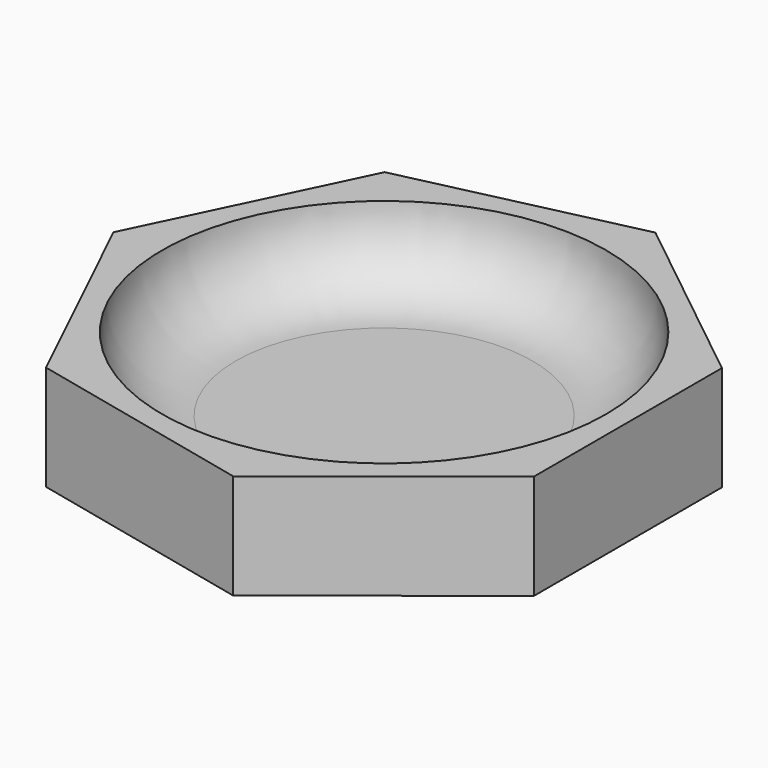
from build123d import *

# Parameters (mm, degrees)
F1_DEPTH = 25.4
F2_R     = 53.6748278482
F3_DEPTH = 17.78
F4_R     = 17.77999


# Not quite as in the source:
# - a fillet or chamfer is up to 0.001 mm smaller than in the source, because OpenCascade refuses the exact size


with BuildPart() as f1:
    # F0 (on Top) → F1 (new body)
    with BuildSketch(Plane.XY):
        Polygon((58.9595362544, -28.3934161968), (58.9595362544, 28.3934161968), (14.5618028995, 63.799427074), (-40.8012650454, 51.1631680934), (-65.440148217, 0), (-40.8012650454, -51.1631680934), (14.5618028995, -63.799427074), align=None)
    extrude(amount=F1_DEPTH)

    # F2 (on face) → F3 (cut)
    with BuildSketch(Plane.XY.offset(25.4)):
        Circle(F2_R)
    extrude(amount=-F3_DEPTH, mode=Mode.SUBTRACT)

    # F4 (radius 17.78 in the source; OpenCascade refuses exactly that, so slightly less here)
    f4_edges = [f1.edges().sort_by_distance(p)[0] for p in [
        (-53.674828, 0, 7.62),
    ]]
    fillet(f4_edges, radius=F4_R)


solid = f1.part
